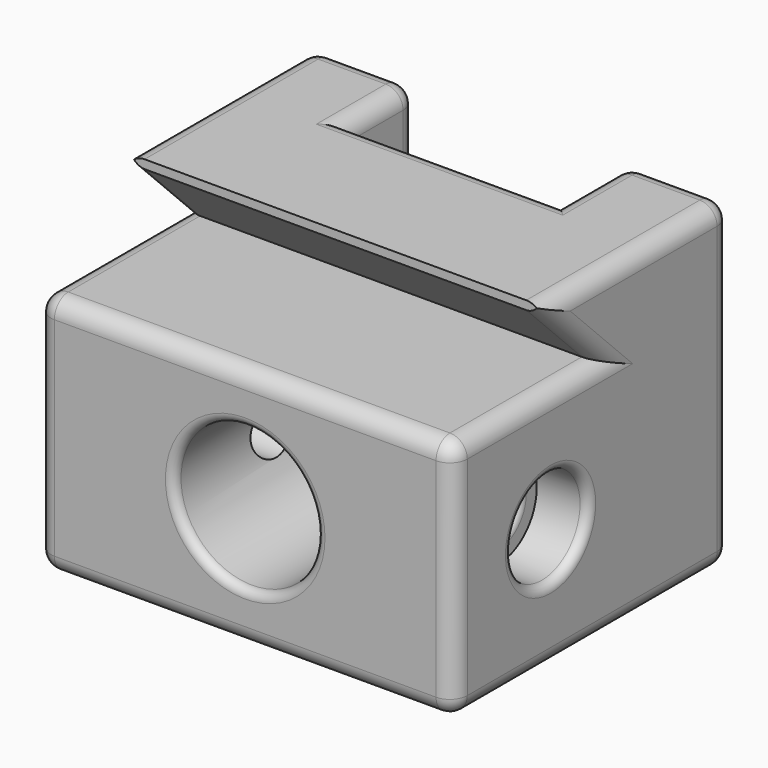
from build123d import *

# Parameters (mm, degrees)
F1_DEPTH       = 18.5
F2_R           = 1.5
F3_DEPTH       = 25
F4_R           = 2.75
F4_R_2         = 1.5
F5_DEPTH       = 3
F7_DEPTH       = 10.5
F8_R           = 4.1
F9_DEPTH       = 25
F10_T1_DEPTH   = 15
F10_T3_DEPTH   = 16.5
F10_T5_DEPTH   = 12
F10_T7_DEPTH   = 18
F10_T9_DEPTH   = 3.9
F10_T11_DEPTH  = 4
F10_T13_DEPTH  = 12.2
F10_T15_DEPTH  = 3.9
F10_T17_DEPTH  = 22
F10_T19_DEPTH  = 2.75
F10_T21_DEPTH  = 5.5
F10_S25_W      = 1
F10_S25_H      = 1
F10_T26_DEPTH  = 1
F10_S31_W      = 1
F10_S31_H      = 1
F10_T32_DEPTH  = 1
F10_S37_W      = 1
F10_S37_H      = 1
F10_T38_DEPTH  = 1
F10_S43_W      = 1
F10_S43_H      = 1
F10_T44_DEPTH  = 1
F10_S49_W      = 1
F10_S49_H      = 1
F10_T50_DEPTH  = 1
F10_S55_W      = 1
F10_S55_H      = 1
F10_T56_DEPTH  = 1
F10_S61_W      = 1
F10_S61_H      = 1
F10_T62_DEPTH  = 1
F10_S67_W      = 1
F10_S67_H      = 1
F10_T68_DEPTH  = 1
F10_S73_W      = 1
F10_S73_H      = 1
F10_T74_DEPTH  = 1
F10_S79_W      = 1
F10_S79_H      = 1
F10_T80_DEPTH  = 1
F10_S85_W      = 1
F10_S85_H      = 1
F10_T86_DEPTH  = 1
F10_S91_W      = 1
F10_S91_H      = 1
F10_T92_DEPTH  = 1
F10_T98_DEPTH  = 12
F10_T103_DEPTH = 10.6568542495
F10_T108_DEPTH = 12
F10_T113_DEPTH = 10.6568542495
F10_T119_DEPTH = 12
F10_T123_DEPTH = 10.6568542495
F10_T130_DEPTH = 14.7
F10_T134_DEPTH = 6.5
F10_T141_DEPTH = 6.5
F10_T145_DEPTH = 14.7
F10_T152_DEPTH = 6.5
F10_T156_DEPTH = 14.7
F10_T163_DEPTH = 14.7
F10_T167_DEPTH = 6.5
F10_T174_DEPTH = 8
F10_T178_DEPTH = 5.25
F10_T185_DEPTH = 8
F10_T189_DEPTH = 5.25
F10_T196_DEPTH = 8
F10_T200_DEPTH = 5.25
F10_T207_DEPTH = 5.25
F10_T211_DEPTH = 8
F10_T218_DEPTH = 12
F10_T222_DEPTH = 10.6568542495
F11_R          = 0.5


# Not quite as in the source:
# - a fillet or chamfer that OpenCascade refuses, or shapes differently, is made with other operations: its cross-section is extruded or revolved along the edge and cut away or added


with BuildPart() as f1:
    # F0 (on Top) → F1 (new body)
    with BuildSketch(Plane.XY):
        Polygon((12, -10), (12, 10), (6.1, 10), (6.1, 5), (-6.1, 5), (-6.1, 10), (-12, 10), (-12, -10), align=None)
    extrude(amount=F1_DEPTH)

    # F2 (on face) → F3 (cut)
    with BuildSketch(Plane(origin=(-12, 0, 0), x_dir=(0, -1, 0), z_dir=(-1, 0, 0))):
        Polygon((-0.5, 14), (10, 14), (10, 18.5), (3.5, 18.5), (3.5, 18), align=None)
        with Locations((3, 7)):
            Circle(F2_R)
    extrude(amount=-F3_DEPTH, mode=Mode.SUBTRACT)

    # F4 (on face) → F5 (cut)
    with BuildSketch(Plane.YZ.offset(12)):
        with Locations((-3, 7)):
            Circle(F4_R)
        with Locations((-3, 7)):
            Circle(F4_R_2, mode=Mode.SUBTRACT)
    extrude(amount=-F5_DEPTH, mode=Mode.SUBTRACT)

    # F6 (on face) → F7 (cut)
    with BuildSketch(Plane(origin=(0, 0, 0), x_dir=(1, 0, 0), z_dir=(0, 0, -1))):
        Polygon((-7.05, 0.25), (-7.05, 3), (-7.05, 5.75), (-9.8, 5.75), (-9.8, 0.25), align=None)
    extrude(amount=-F7_DEPTH, mode=Mode.SUBTRACT)

    # F8 (on face) → F9 (cut)
    with BuildSketch(Plane.XZ.offset(10)):
        with Locations((0, 7)):
            Circle(F8_R)
    extrude(amount=-F9_DEPTH, mode=Mode.SUBTRACT)

    # F10: fillet of radius 1 on 30 edges, made by hand

    # F10_s2 → F10_t1 (cut)
    with BuildSketch(Plane.XZ.offset(-9)):
        with BuildLine():
            ThreePointArc((12, 17.5), (11.7071067812, 18.2071067812), (11, 18.5))
            Line((11, 18.5), (12, 18.5))
            Line((12, 18.5), (12, 17.5))
        make_face()
        with BuildLine():
            ThreePointArc((-11, 18.5), (-11.7071067812, 18.2071067812), (-12, 17.5))
            Line((-12, 17.5), (-12, 18.5))
            Line((-12, 18.5), (-11, 18.5))
        make_face()
    extrude(amount=F10_T1_DEPTH, mode=Mode.SUBTRACT)

    # F10_s4 → F10_t3 (cut)
    with BuildSketch(Plane.XY.offset(1)):
        with BuildLine():
            ThreePointArc((12, 9), (11.7071067812, 9.7071067812), (11, 10))
            Line((11, 10), (12, 10))
            Line((12, 10), (12, 9))
        make_face()
        with BuildLine():
            ThreePointArc((-7.1, 10), (-6.3928932188, 9.7071067812), (-6.1, 9))
            Line((-6.1, 9), (-6.1, 10))
            Line((-6.1, 10), (-7.1, 10))
        make_face()
        with BuildLine():
            ThreePointArc((7.1, 10), (6.3928932188, 9.7071067812), (6.1, 9))
            Line((6.1, 9), (6.1, 10))
            Line((6.1, 10), (7.1, 10))
        make_face()
        with BuildLine():
            ThreePointArc((-12, 9), (-11.7071067812, 9.7071067812), (-11, 10))
            Line((-11, 10), (-12, 10))
            Line((-12, 10), (-12, 9))
        make_face()
    extrude(amount=F10_T3_DEPTH, mode=Mode.SUBTRACT)

    # F10_s6 → F10_t5 (cut)
    with BuildSketch(Plane.XY.offset(1)):
        with BuildLine():
            ThreePointArc((12, -9), (11.7071067812, -9.7071067812), (11, -10))
            Line((11, -10), (12, -10))
            Line((12, -10), (12, -9))
        make_face()
        with BuildLine():
            ThreePointArc((-11, -10), (-11.7071067812, -9.7071067812), (-12, -9))
            Line((-12, -9), (-12, -10))
            Line((-12, -10), (-11, -10))
        make_face()
    extrude(amount=F10_T5_DEPTH, mode=Mode.SUBTRACT)

    # F10_s8 → F10_t7 (cut)
    with BuildSketch(Plane.XZ.offset(-9)):
        with BuildLine():
            ThreePointArc((12, 1), (11.7071067812, 0.2928932188), (11, 0))
            Line((11, 0), (12, 0))
            Line((12, 0), (12, 1))
        make_face()
        with BuildLine():
            ThreePointArc((-11, 0), (-11.7071067812, 0.2928932188), (-12, 1))
            Line((-12, 1), (-12, 0))
            Line((-12, 0), (-11, 0))
        make_face()
    extrude(amount=F10_T7_DEPTH, mode=Mode.SUBTRACT)

    # F10_s10 → F10_t9 (cut)
    with BuildSketch(Plane.YZ.offset(7.1)):
        with BuildLine():
            ThreePointArc((10, 17.5), (9.7071067812, 18.2071067812), (9, 18.5))
            Line((9, 18.5), (10, 18.5))
            Line((10, 18.5), (10, 17.5))
        make_face()
        with BuildLine():
            ThreePointArc((9, 0), (9.7071067812, 0.2928932188), (10, 1))
            Line((10, 1), (10, 0))
            Line((10, 0), (9, 0))
        make_face()
    extrude(amount=F10_T9_DEPTH, mode=Mode.SUBTRACT)

    # F10_s12 → F10_t11 (cut)
    with BuildSketch(Plane.XZ.offset(-9)):
        with BuildLine():
            ThreePointArc((7.1, 18.5), (6.3928932188, 18.2071067812), (6.1, 17.5))
            Line((6.1, 17.5), (6.1, 18.5))
            Line((6.1, 18.5), (7.1, 18.5))
        make_face()
        with BuildLine():
            ThreePointArc((-7.1, 18.5), (-6.3928932188, 18.2071067812), (-6.1, 17.5))
            Line((-6.1, 17.5), (-6.1, 18.5))
            Line((-6.1, 18.5), (-7.1, 18.5))
        make_face()
        with BuildLine():
            ThreePointArc((7.1, 0), (6.3928932188, 0.2928932188), (6.1, 1))
            Line((6.1, 1), (6.1, 0))
            Line((6.1, 0), (7.1, 0))
        make_face()
        with BuildLine():
            ThreePointArc((-7.1, 0), (-6.3928932188, 0.2928932188), (-6.1, 1))
            Line((-6.1, 1), (-6.1, 0))
            Line((-6.1, 0), (-7.1, 0))
        make_face()
    extrude(amount=F10_T11_DEPTH, mode=Mode.SUBTRACT)

    # F10_s14 → F10_t13 (cut)
    with BuildSketch(Plane.YZ.offset(-6.1)):
        with BuildLine():
            ThreePointArc((4, 18.5), (4.7071067812, 18.2071067812), (5, 17.5))
            Line((5, 17.5), (5, 18.5))
            Line((5, 18.5), (4, 18.5))
        make_face()
        with BuildLine():
            ThreePointArc((4, 0), (4.7071067812, 0.2928932188), (5, 1))
            Line((5, 1), (5, 0))
            Line((5, 0), (4, 0))
        make_face()
    extrude(amount=F10_T13_DEPTH, mode=Mode.SUBTRACT)

    # F10_s16 → F10_t15 (cut)
    with BuildSketch(Plane.YZ.offset(-11)):
        with BuildLine():
            ThreePointArc((9, 18.5), (9.7071067812, 18.2071067812), (10, 17.5))
            Line((10, 17.5), (10, 18.5))
            Line((10, 18.5), (9, 18.5))
        make_face()
        with BuildLine():
            ThreePointArc((9, 0), (9.7071067812, 0.2928932188), (10, 1))
            Line((10, 1), (10, 0))
            Line((10, 0), (9, 0))
        make_face()
    extrude(amount=F10_T15_DEPTH, mode=Mode.SUBTRACT)

    # F10_s18 → F10_t17 (cut)
    with BuildSketch(Plane.YZ.offset(-11)):
        with BuildLine():
            ThreePointArc((-9, 0), (-9.7071067812, 0.2928932188), (-10, 1))
            Line((-10, 1), (-10, 0))
            Line((-10, 0), (-9, 0))
        make_face()
        with BuildLine():
            ThreePointArc((-10, 13), (-9.7071067812, 13.7071067812), (-9, 14))
            Line((-9, 14), (-10, 14))
            Line((-10, 14), (-10, 13))
        make_face()
    extrude(amount=F10_T17_DEPTH, mode=Mode.SUBTRACT)

    # F10_s20 → F10_t19 (cut)
    with BuildSketch(Plane.YZ.offset(-9.8)):
        with BuildLine():
            ThreePointArc((-6.75, 0), (-6.0428932188, 0.2928932188), (-5.75, 1))
            Line((-5.75, 1), (-5.75, 0))
            Line((-5.75, 0), (-6.75, 0))
        make_face()
        with BuildLine():
            ThreePointArc((0.75, 0), (0.0428932188, 0.2928932188), (-0.25, 1))
            Line((-0.25, 1), (-0.25, 0))
            Line((-0.25, 0), (0.75, 0))
        make_face()
    extrude(amount=F10_T19_DEPTH, mode=Mode.SUBTRACT)

    # F10_s22 → F10_t21 (cut)
    with BuildSketch(Plane.XZ.offset(0.25)):
        with BuildLine():
            ThreePointArc((-6.05, 0), (-6.7571067812, 0.2928932188), (-7.05, 1))
            Line((-7.05, 1), (-7.05, 0))
            Line((-7.05, 0), (-6.05, 0))
        make_face()
        with BuildLine():
            ThreePointArc((-10.8, 0), (-10.0928932188, 0.2928932188), (-9.8, 1))
            Line((-9.8, 1), (-9.8, 0))
            Line((-9.8, 0), (-10.8, 0))
        make_face()
    extrude(amount=F10_T21_DEPTH, mode=Mode.SUBTRACT)


with BuildPart() as f10_tool24:
    # F10_s25 → F10_t26 (new body)
    with BuildSketch(Plane.YZ.offset(11)):
        with Locations((-9.5, 13.5)):
            Rectangle(F10_S25_W, F10_S25_H)
    extrude(amount=F10_T26_DEPTH)

    # F10_s27 → F10_t28 (revolve, cut)
    with BuildSketch(Plane(origin=(11, -9, 13), x_dir=(0, 0.7071067812, -0.7071067812), z_dir=(0, -0.7071067812, -0.7071067812))):
        with BuildLine():
            ThreePointArc((0, -1), (1, 0), (0, 1))
            Line((0, 1), (0, -1))
        make_face()
    revolve(axis=Axis((11, -9, 13), (1, 0, 0)), mode=Mode.SUBTRACT)


with BuildPart() as f1_1:
    add(f1.part)

    # F10_t23: cut F10_tool24
    add(f10_tool24.part, mode=Mode.SUBTRACT)


with BuildPart() as f10_tool30:
    # F10_s31 → F10_t32 (new body)
    with BuildSketch(Plane.YZ.offset(11)):
        with Locations((9.5, 18)):
            Rectangle(F10_S31_W, F10_S31_H)
    extrude(amount=F10_T32_DEPTH)

    # F10_s33 → F10_t34 (revolve, cut)
    with BuildSketch(Plane(origin=(11, 9, 17.5), x_dir=(0, -0.7071067812, -0.7071067812), z_dir=(0, -0.7071067812, 0.7071067812))):
        with BuildLine():
            ThreePointArc((0, -1), (1, 0), (0, 1))
            Line((0, 1), (0, -1))
        make_face()
    revolve(axis=Axis((11, 9, 17.5), (1, 0, 0)), mode=Mode.SUBTRACT)


with BuildPart() as f1_2:
    add(f1_1.part)

    # F10_t29: cut F10_tool30
    add(f10_tool30.part, mode=Mode.SUBTRACT)


with BuildPart() as f10_tool36:
    # F10_s37 → F10_t38 (new body)
    with BuildSketch(Plane.YZ.offset(11)):
        with Locations((9.5, 0.5)):
            Rectangle(F10_S37_W, F10_S37_H)
    extrude(amount=F10_T38_DEPTH)

    # F10_s39 → F10_t40 (revolve, cut)
    with BuildSketch(Plane(origin=(11, 9, 1), x_dir=(0, -0.7071067812, 0.7071067812), z_dir=(0, 0.7071067812, 0.7071067812))):
        with BuildLine():
            ThreePointArc((0, -1), (1, 0), (0, 1))
            Line((0, 1), (0, -1))
        make_face()
    revolve(axis=Axis((11, 9, 1), (1, 0, 0)), mode=Mode.SUBTRACT)


with BuildPart() as f1_3:
    add(f1_2.part)

    # F10_t35: cut F10_tool36
    add(f10_tool36.part, mode=Mode.SUBTRACT)


with BuildPart() as f10_tool42:
    # F10_s43 → F10_t44 (new body)
    with BuildSketch(Plane.YZ.offset(11)):
        with Locations((-9.5, 0.5)):
            Rectangle(F10_S43_W, F10_S43_H)
    extrude(amount=F10_T44_DEPTH)

    # F10_s45 → F10_t46 (revolve, cut)
    with BuildSketch(Plane(origin=(11, -9, 1), x_dir=(0, 0.7071067812, 0.7071067812), z_dir=(0, 0.7071067812, -0.7071067812))):
        with BuildLine():
            ThreePointArc((0, -1), (1, 0), (0, 1))
            Line((0, 1), (0, -1))
        make_face()
    revolve(axis=Axis((11, -9, 1), (1, 0, 0)), mode=Mode.SUBTRACT)


with BuildPart() as f1_4:
    add(f1_3.part)

    # F10_t41: cut F10_tool42
    add(f10_tool42.part, mode=Mode.SUBTRACT)


with BuildPart() as f10_tool48:
    # F10_s49 → F10_t50 (new body)
    with BuildSketch(Plane.YZ.offset(7.1)):
        with Locations((9.5, 18)):
            Rectangle(F10_S49_W, F10_S49_H)
    extrude(amount=-F10_T50_DEPTH)

    # F10_s51 → F10_t52 (revolve, cut)
    with BuildSketch(Plane(origin=(7.1, 9, 17.5), x_dir=(0, -0.7071067812, -0.7071067812), z_dir=(0, 0.7071067812, -0.7071067812))):
        with BuildLine():
            ThreePointArc((0, -1), (1, 0), (0, 1))
            Line((0, 1), (0, -1))
        make_face()
    revolve(axis=Axis((7.1, 9, 17.5), (-1, 0, 0)), mode=Mode.SUBTRACT)


with BuildPart() as f1_5:
    add(f1_4.part)

    # F10_t47: cut F10_tool48
    add(f10_tool48.part, mode=Mode.SUBTRACT)


with BuildPart() as f10_tool54:
    # F10_s55 → F10_t56 (new body)
    with BuildSketch(Plane.YZ.offset(-7.1)):
        with Locations((9.5, 18)):
            Rectangle(F10_S55_W, F10_S55_H)
    extrude(amount=F10_T56_DEPTH)

    # F10_s57 → F10_t58 (revolve, cut)
    with BuildSketch(Plane(origin=(-7.1, 9, 17.5), x_dir=(0, -0.7071067812, -0.7071067812), z_dir=(0, -0.7071067812, 0.7071067812))):
        with BuildLine():
            ThreePointArc((0, -1), (1, 0), (0, 1))
            Line((0, 1), (0, -1))
        make_face()
    revolve(axis=Axis((-7.1, 9, 17.5), (1, 0, 0)), mode=Mode.SUBTRACT)


with BuildPart() as f1_6:
    add(f1_5.part)

    # F10_t53: cut F10_tool54
    add(f10_tool54.part, mode=Mode.SUBTRACT)


with BuildPart() as f10_tool60:
    # F10_s61 → F10_t62 (new body)
    with BuildSketch(Plane.YZ.offset(-11)):
        with Locations((9.5, 18)):
            Rectangle(F10_S61_W, F10_S61_H)
    extrude(amount=-F10_T62_DEPTH)

    # F10_s63 → F10_t64 (revolve, cut)
    with BuildSketch(Plane(origin=(-11, 9, 17.5), x_dir=(0, -0.7071067812, -0.7071067812), z_dir=(0, 0.7071067812, -0.7071067812))):
        with BuildLine():
            ThreePointArc((0, -1), (1, 0), (0, 1))
            Line((0, 1), (0, -1))
        make_face()
    revolve(axis=Axis((-11, 9, 17.5), (-1, 0, 0)), mode=Mode.SUBTRACT)


with BuildPart() as f1_7:
    add(f1_6.part)

    # F10_t59: cut F10_tool60
    add(f10_tool60.part, mode=Mode.SUBTRACT)


with BuildPart() as f10_tool66:
    # F10_s67 → F10_t68 (new body)
    with BuildSketch(Plane.XY.offset(1)):
        with Locations((-6.6, 9.5)):
            Rectangle(F10_S67_W, F10_S67_H)
    extrude(amount=-F10_T68_DEPTH)

    # F10_s69 → F10_t70 (revolve, cut)
    with BuildSketch(Plane(origin=(-7.1, 9, 1), x_dir=(-0.7071067812, -0.7071067812, 0), z_dir=(0.7071067812, -0.7071067812, 0))):
        with BuildLine():
            ThreePointArc((0, -1), (1, 0), (0, 1))
            Line((0, 1), (0, -1))
        make_face()
    revolve(axis=Axis((-7.1, 9, 1), (0, 0, -1)), mode=Mode.SUBTRACT)


with BuildPart() as f1_8:
    add(f1_7.part)

    # F10_t65: cut F10_tool66
    add(f10_tool66.part, mode=Mode.SUBTRACT)


with BuildPart() as f10_tool72:
    # F10_s73 → F10_t74 (new body)
    with BuildSketch(Plane.XY.offset(1)):
        with Locations((6.6, 9.5)):
            Rectangle(F10_S73_W, F10_S73_H)
    extrude(amount=-F10_T74_DEPTH)

    # F10_s75 → F10_t76 (revolve, cut)
    with BuildSketch(Plane(origin=(7.1, 9, 1), x_dir=(0.7071067812, -0.7071067812, 0), z_dir=(0.7071067812, 0.7071067812, 0))):
        with BuildLine():
            ThreePointArc((0, -1), (1, 0), (0, 1))
            Line((0, 1), (0, -1))
        make_face()
    revolve(axis=Axis((7.1, 9, 1), (0, 0, -1)), mode=Mode.SUBTRACT)


with BuildPart() as f1_9:
    add(f1_8.part)

    # F10_t71: cut F10_tool72
    add(f10_tool72.part, mode=Mode.SUBTRACT)


with BuildPart() as f10_tool78:
    # F10_s79 → F10_t80 (new body)
    with BuildSketch(Plane.YZ.offset(-11)):
        with Locations((9.5, 0.5)):
            Rectangle(F10_S79_W, F10_S79_H)
    extrude(amount=-F10_T80_DEPTH)

    # F10_s81 → F10_t82 (revolve, cut)
    with BuildSketch(Plane(origin=(-11, 9, 1), x_dir=(0, -0.7071067812, 0.7071067812), z_dir=(0, -0.7071067812, -0.7071067812))):
        with BuildLine():
            ThreePointArc((0, -1), (1, 0), (0, 1))
            Line((0, 1), (0, -1))
        make_face()
    revolve(axis=Axis((-11, 9, 1), (-1, 0, 0)), mode=Mode.SUBTRACT)


with BuildPart() as f1_10:
    add(f1_9.part)

    # F10_t77: cut F10_tool78
    add(f10_tool78.part, mode=Mode.SUBTRACT)


with BuildPart() as f10_tool84:
    # F10_s85 → F10_t86 (new body)
    with BuildSketch(Plane.XY.offset(1)):
        with Locations((-11.5, -9.5)):
            Rectangle(F10_S85_W, F10_S85_H)
    extrude(amount=-F10_T86_DEPTH)

    # F10_s87 → F10_t88 (revolve, cut)
    with BuildSketch(Plane(origin=(-11, -9, 1), x_dir=(0.7071067812, 0.7071067812, 0), z_dir=(-0.7071067812, 0.7071067812, 0))):
        with BuildLine():
            ThreePointArc((0, -1), (1, 0), (0, 1))
            Line((0, 1), (0, -1))
        make_face()
    revolve(axis=Axis((-11, -9, 1), (0, 0, -1)), mode=Mode.SUBTRACT)


with BuildPart() as f1_11:
    add(f1_10.part)

    # F10_t83: cut F10_tool84
    add(f10_tool84.part, mode=Mode.SUBTRACT)


with BuildPart() as f10_tool90:
    # F10_s91 → F10_t92 (new body)
    with BuildSketch(Plane.YZ.offset(-11)):
        with Locations((-9.5, 13.5)):
            Rectangle(F10_S91_W, F10_S91_H)
    extrude(amount=-F10_T92_DEPTH)

    # F10_s93 → F10_t94 (revolve, cut)
    with BuildSketch(Plane(origin=(-11, -9, 13), x_dir=(0, 0.7071067812, -0.7071067812), z_dir=(0, 0.7071067812, 0.7071067812))):
        with BuildLine():
            ThreePointArc((0, -1), (1, 0), (0, 1))
            Line((0, 1), (0, -1))
        make_face()
    revolve(axis=Axis((-11, -9, 13), (-1, 0, 0)), mode=Mode.SUBTRACT)


with BuildPart() as f1_12:
    add(f1_11.part)

    # F10_t89: cut F10_tool90
    add(f10_tool90.part, mode=Mode.SUBTRACT)


with BuildPart() as f10_tool96:
    # F10_s97 → F10_t98 (new body)
    with BuildSketch(Plane.XZ.offset(-3)):
        with BuildLine():
            ThreePointArc((12, 13), (11.7071067812, 13.7071067812), (11, 14))
            Line((11, 14), (12, 14))
            Line((12, 14), (12, 13))
        make_face()
    extrude(amount=F10_T98_DEPTH)

    split(bisect_by=Plane(origin=(0, 7.25, 7.25), x_dir=(1, 0, 0), z_dir=(0, -0.7071067812, -0.7071067812)), keep=Keep.TOP)


with BuildPart() as f1_13:
    add(f1_12.part)

    # F10_t95: cut F10_tool96
    add(f10_tool96.part, mode=Mode.SUBTRACT)


with BuildPart() as f10_tool101:
    # F10_s102 → F10_t103 (new body)
    with BuildSketch(Plane(origin=(0, -12.517766953, 12.517766953), x_dir=(1, 0, 0), z_dir=(0, 0.7071067812, -0.7071067812))):
        with BuildLine():
            ThreePointArc((12, -11.2530483272), (11.7071067812, -10.545941546), (11, -10.2530483272))
            Line((11, -10.2530483272), (12, -10.2530483272))
            Line((12, -10.2530483272), (12, -11.2530483272))
        make_face()
    extrude(amount=F10_T103_DEPTH)

    split(bisect_by=Plane.XY.offset(14), keep=Keep.TOP)


with BuildPart() as f1_14:
    add(f1_13.part)

    # F10_t100: cut F10_tool101
    add(f10_tool101.part, mode=Mode.SUBTRACT)


with BuildPart() as f10_tool106:
    # F10_s107 → F10_t108 (new body)
    with BuildSketch(Plane.XZ.offset(-3)):
        with BuildLine():
            ThreePointArc((-11, 14), (-11.7071067812, 13.7071067812), (-12, 13))
            Line((-12, 13), (-12, 14))
            Line((-12, 14), (-11, 14))
        make_face()
    extrude(amount=F10_T108_DEPTH)

    split(bisect_by=Plane(origin=(0, 7.25, 7.25), x_dir=(1, 0, 0), z_dir=(0, -0.7071067812, -0.7071067812)), keep=Keep.TOP)


with BuildPart() as f1_15:
    add(f1_14.part)

    # F10_t105: cut F10_tool106
    add(f10_tool106.part, mode=Mode.SUBTRACT)


with BuildPart() as f10_tool111:
    # F10_s112 → F10_t113 (new body)
    with BuildSketch(Plane(origin=(0, -12.517766953, 12.517766953), x_dir=(1, 0, 0), z_dir=(0, 0.7071067812, -0.7071067812))):
        with BuildLine():
            ThreePointArc((-11, -10.2530483272), (-11.7071067812, -10.545941546), (-12, -11.2530483272))
            Line((-12, -11.2530483272), (-12, -10.2530483272))
            Line((-12, -10.2530483272), (-11, -10.2530483272))
        make_face()
    extrude(amount=F10_T113_DEPTH)

    split(bisect_by=Plane.XY.offset(14), keep=Keep.TOP)


with BuildPart() as f1_16:
    add(f1_15.part)

    # F10_t110: cut F10_tool111
    add(f10_tool111.part, mode=Mode.SUBTRACT)


with BuildPart() as f10_tool117:
    # F10_s118 → F10_t119 (new body)
    with BuildSketch(Plane.XZ.offset(-3)):
        with BuildLine():
            ThreePointArc((12, 13), (11.7071067812, 13.7071067812), (11, 14))
            Line((11, 14), (12, 14))
            Line((12, 14), (12, 13))
        make_face()
    extrude(amount=F10_T119_DEPTH)

    split(bisect_by=Plane(origin=(0, 7.25, 7.25), x_dir=(1, 0, 0), z_dir=(0, 0.7071067812, 0.7071067812)), keep=Keep.TOP)


with BuildPart() as f10_tool121:
    # F10_s122 → F10_t123 (new body)
    with BuildSketch(Plane(origin=(0, -12.517766953, 12.517766953), x_dir=(1, 0, 0), z_dir=(0, 0.7071067812, -0.7071067812))):
        with BuildLine():
            ThreePointArc((12, -11.2530483272), (11.7071067812, -10.545941546), (11, -10.2530483272))
            Line((11, -10.2530483272), (12, -10.2530483272))
            Line((12, -10.2530483272), (12, -11.2530483272))
        make_face()
    extrude(amount=F10_T123_DEPTH)

    split(bisect_by=Plane.XY.offset(14), keep=Keep.BOTTOM)


with BuildPart() as f10_tool117_1:
    add(f10_tool117.part)

    # F10_t125: intersect F10_tool121
    add(f10_tool121.part, mode=Mode.INTERSECT)


with BuildPart() as f1_17:
    add(f1_16.part)

    # F10_t115: cut F10_tool117
    add(f10_tool117_1.part, mode=Mode.SUBTRACT)


with BuildPart() as f10_tool128:
    # F10_s129 → F10_t130 (new body)
    with BuildSketch(Plane.YZ.offset(8.6)):
        with BuildLine():
            ThreePointArc((4, 18.5), (4.7071067812, 18.2071067812), (5, 17.5))
            Line((5, 17.5), (5, 18.5))
            Line((5, 18.5), (4, 18.5))
        make_face()
    extrude(amount=-F10_T130_DEPTH)

    split(bisect_by=Plane.YZ.offset(6.1), keep=Keep.TOP)


with BuildPart() as f10_tool132:
    # F10_s133 → F10_t134 (new body)
    with BuildSketch(Plane.XZ.offset(-9)):
        with BuildLine():
            ThreePointArc((7.1, 18.5), (6.3928932188, 18.2071067812), (6.1, 17.5))
            Line((6.1, 17.5), (6.1, 18.5))
            Line((6.1, 18.5), (7.1, 18.5))
        make_face()
    extrude(amount=F10_T134_DEPTH)

    split(bisect_by=Plane.XZ.offset(-5), keep=Keep.TOP)


with BuildPart() as f10_tool128_1:
    add(f10_tool128.part)

    # F10_t136: intersect F10_tool132
    add(f10_tool132.part, mode=Mode.INTERSECT)


with BuildPart() as f1_18:
    add(f1_17.part)

    # F10_t126: cut F10_tool128
    add(f10_tool128_1.part, mode=Mode.SUBTRACT)


with BuildPart() as f10_tool139:
    # F10_s140 → F10_t141 (new body)
    with BuildSketch(Plane.XZ.offset(-2.5)):
        with BuildLine():
            ThreePointArc((-7.1, 18.5), (-6.3928932188, 18.2071067812), (-6.1, 17.5))
            Line((-6.1, 17.5), (-6.1, 18.5))
            Line((-6.1, 18.5), (-7.1, 18.5))
        make_face()
    extrude(amount=-F10_T141_DEPTH)

    split(bisect_by=Plane.XZ.offset(-5), keep=Keep.TOP)


with BuildPart() as f10_tool143:
    # F10_s144 → F10_t145 (new body)
    with BuildSketch(Plane.YZ.offset(6.1)):
        with BuildLine():
            ThreePointArc((4, 18.5), (4.7071067812, 18.2071067812), (5, 17.5))
            Line((5, 17.5), (5, 18.5))
            Line((5, 18.5), (4, 18.5))
        make_face()
    extrude(amount=-F10_T145_DEPTH)

    split(bisect_by=Plane.YZ.offset(-6.1), keep=Keep.BOTTOM)


with BuildPart() as f10_tool139_1:
    add(f10_tool139.part)

    # F10_t147: intersect F10_tool143
    add(f10_tool143.part, mode=Mode.INTERSECT)


with BuildPart() as f1_19:
    add(f1_18.part)

    # F10_t137: cut F10_tool139
    add(f10_tool139_1.part, mode=Mode.SUBTRACT)


with BuildPart() as f10_tool150:
    # F10_s151 → F10_t152 (new body)
    with BuildSketch(Plane.XZ.offset(-9)):
        with BuildLine():
            ThreePointArc((7.1, 0), (6.3928932188, 0.2928932188), (6.1, 1))
            Line((6.1, 1), (6.1, 0))
            Line((6.1, 0), (7.1, 0))
        make_face()
    extrude(amount=F10_T152_DEPTH)

    split(bisect_by=Plane.XZ.offset(-5), keep=Keep.TOP)


with BuildPart() as f10_tool154:
    # F10_s155 → F10_t156 (new body)
    with BuildSketch(Plane.YZ.offset(8.6)):
        with BuildLine():
            ThreePointArc((4, 0), (4.7071067812, 0.2928932188), (5, 1))
            Line((5, 1), (5, 0))
            Line((5, 0), (4, 0))
        make_face()
    extrude(amount=-F10_T156_DEPTH)

    split(bisect_by=Plane.YZ.offset(6.1), keep=Keep.TOP)


with BuildPart() as f10_tool150_1:
    add(f10_tool150.part)

    # F10_t158: intersect F10_tool154
    add(f10_tool154.part, mode=Mode.INTERSECT)


with BuildPart() as f1_20:
    add(f1_19.part)

    # F10_t148: cut F10_tool150
    add(f10_tool150_1.part, mode=Mode.SUBTRACT)


with BuildPart() as f10_tool161:
    # F10_s162 → F10_t163 (new body)
    with BuildSketch(Plane.YZ.offset(6.1)):
        with BuildLine():
            ThreePointArc((4, 0), (4.7071067812, 0.2928932188), (5, 1))
            Line((5, 1), (5, 0))
            Line((5, 0), (4, 0))
        make_face()
    extrude(amount=-F10_T163_DEPTH)

    split(bisect_by=Plane.YZ.offset(-6.1), keep=Keep.BOTTOM)


with BuildPart() as f10_tool165:
    # F10_s166 → F10_t167 (new body)
    with BuildSketch(Plane.XZ.offset(-2.5)):
        with BuildLine():
            ThreePointArc((-7.1, 0), (-6.3928932188, 0.2928932188), (-6.1, 1))
            Line((-6.1, 1), (-6.1, 0))
            Line((-6.1, 0), (-7.1, 0))
        make_face()
    extrude(amount=-F10_T167_DEPTH)

    split(bisect_by=Plane.XZ.offset(-5), keep=Keep.TOP)


with BuildPart() as f10_tool161_1:
    add(f10_tool161.part)

    # F10_t169: intersect F10_tool165
    add(f10_tool165.part, mode=Mode.INTERSECT)


with BuildPart() as f1_21:
    add(f1_20.part)

    # F10_t159: cut F10_tool161
    add(f10_tool161_1.part, mode=Mode.SUBTRACT)


with BuildPart() as f10_tool172:
    # F10_s173 → F10_t174 (new body)
    with BuildSketch(Plane.XZ.offset(8.25)):
        with BuildLine():
            ThreePointArc((-6.05, 0), (-6.7571067812, 0.2928932188), (-7.05, 1))
            Line((-7.05, 1), (-7.05, 0))
            Line((-7.05, 0), (-6.05, 0))
        make_face()
    extrude(amount=-F10_T174_DEPTH)

    split(bisect_by=Plane.XZ.offset(5.75), keep=Keep.TOP)


with BuildPart() as f10_tool176:
    # F10_s177 → F10_t178 (new body)
    with BuildSketch(Plane.YZ.offset(-4.55)):
        with BuildLine():
            ThreePointArc((-6.75, 0), (-6.0428932188, 0.2928932188), (-5.75, 1))
            Line((-5.75, 1), (-5.75, 0))
            Line((-5.75, 0), (-6.75, 0))
        make_face()
    extrude(amount=-F10_T178_DEPTH)

    split(bisect_by=Plane.YZ.offset(-7.05), keep=Keep.TOP)


with BuildPart() as f10_tool172_1:
    add(f10_tool172.part)

    # F10_t180: intersect F10_tool176
    add(f10_tool176.part, mode=Mode.INTERSECT)


with BuildPart() as f1_22:
    add(f1_21.part)

    # F10_t170: cut F10_tool172
    add(f10_tool172_1.part, mode=Mode.SUBTRACT)


with BuildPart() as f10_tool183:
    # F10_s184 → F10_t185 (new body)
    with BuildSketch(Plane.XZ.offset(8.25)):
        with BuildLine():
            ThreePointArc((-10.8, 0), (-10.0928932188, 0.2928932188), (-9.8, 1))
            Line((-9.8, 1), (-9.8, 0))
            Line((-9.8, 0), (-10.8, 0))
        make_face()
    extrude(amount=-F10_T185_DEPTH)

    split(bisect_by=Plane.XZ.offset(5.75), keep=Keep.TOP)


with BuildPart() as f10_tool187:
    # F10_s188 → F10_t189 (new body)
    with BuildSketch(Plane.YZ.offset(-7.05)):
        with BuildLine():
            ThreePointArc((-6.75, 0), (-6.0428932188, 0.2928932188), (-5.75, 1))
            Line((-5.75, 1), (-5.75, 0))
            Line((-5.75, 0), (-6.75, 0))
        make_face()
    extrude(amount=-F10_T189_DEPTH)

    split(bisect_by=Plane.YZ.offset(-9.8), keep=Keep.BOTTOM)


with BuildPart() as f10_tool183_1:
    add(f10_tool183.part)

    # F10_t191: intersect F10_tool187
    add(f10_tool187.part, mode=Mode.INTERSECT)


with BuildPart() as f1_23:
    add(f1_22.part)

    # F10_t181: cut F10_tool183
    add(f10_tool183_1.part, mode=Mode.SUBTRACT)


with BuildPart() as f10_tool194:
    # F10_s195 → F10_t196 (new body)
    with BuildSketch(Plane.XZ.offset(5.75)):
        with BuildLine():
            ThreePointArc((-6.05, 0), (-6.7571067812, 0.2928932188), (-7.05, 1))
            Line((-7.05, 1), (-7.05, 0))
            Line((-7.05, 0), (-6.05, 0))
        make_face()
    extrude(amount=-F10_T196_DEPTH)

    split(bisect_by=Plane.XZ.offset(0.25), keep=Keep.BOTTOM)


with BuildPart() as f10_tool198:
    # F10_s199 → F10_t200 (new body)
    with BuildSketch(Plane.YZ.offset(-9.8)):
        with BuildLine():
            ThreePointArc((0.75, 0), (0.0428932188, 0.2928932188), (-0.25, 1))
            Line((-0.25, 1), (-0.25, 0))
            Line((-0.25, 0), (0.75, 0))
        make_face()
    extrude(amount=F10_T200_DEPTH)

    split(bisect_by=Plane.YZ.offset(-7.05), keep=Keep.TOP)


with BuildPart() as f10_tool194_1:
    add(f10_tool194.part)

    # F10_t202: intersect F10_tool198
    add(f10_tool198.part, mode=Mode.INTERSECT)


with BuildPart() as f1_24:
    add(f1_23.part)

    # F10_t192: cut F10_tool194
    add(f10_tool194_1.part, mode=Mode.SUBTRACT)


with BuildPart() as f10_tool205:
    # F10_s206 → F10_t207 (new body)
    with BuildSketch(Plane.YZ.offset(-12.3)):
        with BuildLine():
            ThreePointArc((0.75, 0), (0.0428932188, 0.2928932188), (-0.25, 1))
            Line((-0.25, 1), (-0.25, 0))
            Line((-0.25, 0), (0.75, 0))
        make_face()
    extrude(amount=F10_T207_DEPTH)

    split(bisect_by=Plane.YZ.offset(-9.8), keep=Keep.BOTTOM)


with BuildPart() as f10_tool209:
    # F10_s210 → F10_t211 (new body)
    with BuildSketch(Plane.XZ.offset(5.75)):
        with BuildLine():
            ThreePointArc((-10.8, 0), (-10.0928932188, 0.2928932188), (-9.8, 1))
            Line((-9.8, 1), (-9.8, 0))
            Line((-9.8, 0), (-10.8, 0))
        make_face()
    extrude(amount=-F10_T211_DEPTH)

    split(bisect_by=Plane.XZ.offset(0.25), keep=Keep.BOTTOM)


with BuildPart() as f10_tool205_1:
    add(f10_tool205.part)

    # F10_t213: intersect F10_tool209
    add(f10_tool209.part, mode=Mode.INTERSECT)


with BuildPart() as f1_25:
    add(f1_24.part)

    # F10_t203: cut F10_tool205
    add(f10_tool205_1.part, mode=Mode.SUBTRACT)


with BuildPart() as f10_tool216:
    # F10_s217 → F10_t218 (new body)
    with BuildSketch(Plane.XZ.offset(-3)):
        with BuildLine():
            ThreePointArc((-11, 14), (-11.7071067812, 13.7071067812), (-12, 13))
            Line((-12, 13), (-12, 14))
            Line((-12, 14), (-11, 14))
        make_face()
    extrude(amount=F10_T218_DEPTH)

    split(bisect_by=Plane(origin=(0, 7.25, 7.25), x_dir=(1, 0, 0), z_dir=(0, 0.7071067812, 0.7071067812)), keep=Keep.TOP)


with BuildPart() as f10_tool220:
    # F10_s221 → F10_t222 (new body)
    with BuildSketch(Plane(origin=(0, -12.517766953, 12.517766953), x_dir=(1, 0, 0), z_dir=(0, 0.7071067812, -0.7071067812))):
        with BuildLine():
            ThreePointArc((-11, -10.2530483272), (-11.7071067812, -10.545941546), (-12, -11.2530483272))
            Line((-12, -11.2530483272), (-12, -10.2530483272))
            Line((-12, -10.2530483272), (-11, -10.2530483272))
        make_face()
    extrude(amount=F10_T222_DEPTH)

    split(bisect_by=Plane.XY.offset(14), keep=Keep.BOTTOM)


with BuildPart() as f10_tool216_1:
    add(f10_tool216.part)

    # F10_t224: intersect F10_tool220
    add(f10_tool220.part, mode=Mode.INTERSECT)


with BuildPart() as f1_26:
    add(f1_25.part)

    # F10_t214: cut F10_tool216
    add(f10_tool216_1.part, mode=Mode.SUBTRACT)

    # F11
    f11_edges = [f1_26.edges().sort_by_distance(p)[0] for p in [
        (-4.1, 5, 7),
        (-4.1, -10, 7),
        (12, -5.75, 7),
        (11, 0, 0),
        (9, -1.5, 7),
        (-12, -1.5, 7),
    ]]
    fillet(f11_edges, radius=F11_R)


solid = f1_26.part
